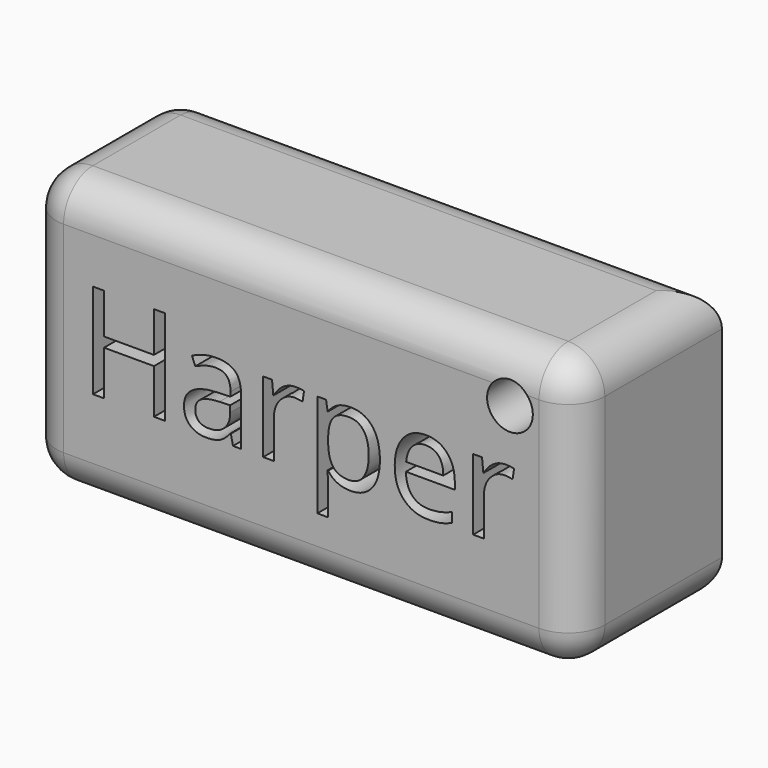
from build123d import *

# Parameters (mm, degrees)
F0_W         = 76.2
F0_H         = 38.1
F1_DEPTH     = 25.4
F3_R         = 5.08
F5_D         = 6.35
F2_TEXT_SIZE = 18.4379380778
F6_DEPTH     = 6.35


# Not quite as in the source:
# - Text() gives the source's letters only with a copy of the font that has no kerning and outlines rounded to 1/6400 em; it was checked with that copy


with BuildPart() as f1:
    # F0 (on Front) → F1 (new body)
    with BuildSketch(Plane.XZ):
        Rectangle(F0_W, F0_H)
    extrude(amount=F1_DEPTH)

    # F3
    f3_edges = [f1.edges().sort_by_distance(p)[0] for p in [
        (0, -25.4, 19.05),
        (38.1, -25.4, 0),
        (38.1, -12.7, 19.05),
        (38.1, -12.7, -19.05),
        (0, -25.4, -19.05),
        (-38.1, -25.4, 0),
        (-38.1, 0, 0),
        (-38.1, -12.7, 19.05),
        (-38.1, -12.7, -19.05),
        (0, 0, 19.05),
        (0, 0, -19.05),
    ]]
    fillet(f3_edges, radius=F3_R)

    # F5 (through all)
    with Locations(Plane.XZ.offset(25.4)):
        with Locations((28.979094699, 11.8943937123)):
            Hole(F5_D / 2)

    # F2 (on face) → F6 (cut)
    with BuildSketch(Plane.XZ.offset(25.4)):
        with Locations((-30.7452617448, -5.5006839232)):
            Text('Harper', F2_TEXT_SIZE, font='Open Sans', text_align=(TextAlign.LEFT, TextAlign.BOTTOM))
    extrude(amount=-F6_DEPTH, mode=Mode.SUBTRACT)


solid = f1.part
